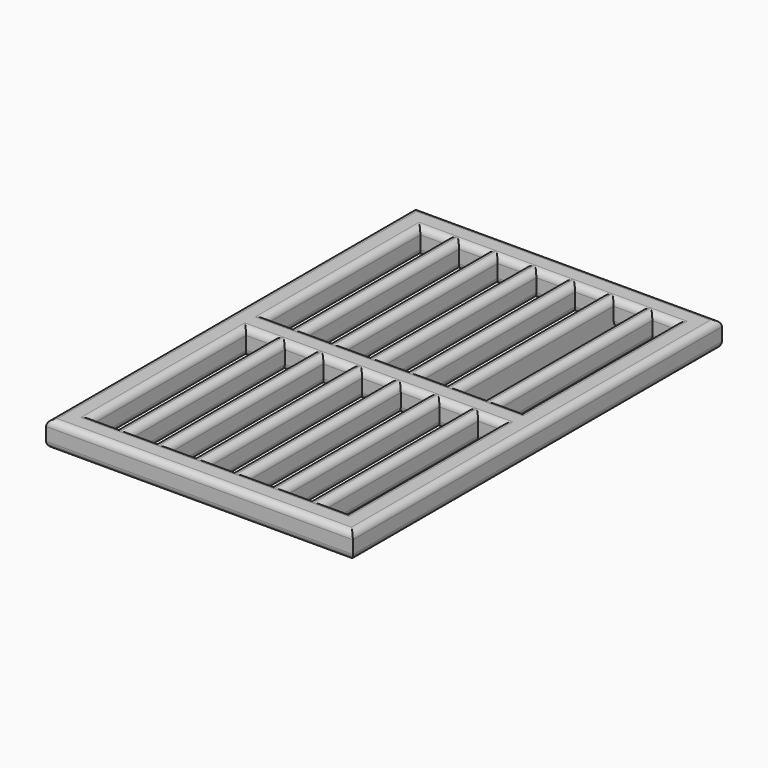
from build123d import *

# Parameters (mm, degrees)
F0_W     = 60.452
F0_H     = 90.932
F0_W_2   = 2.54
F0_H_2   = 37.846
F1_DEPTH = 5.08
F2_R     = 1.26999
F3_R     = 1.26999


# Not quite as in the source:
# - a fillet or chamfer is up to 0.001 mm smaller than in the source, because OpenCascade refuses the exact size


with BuildPart() as f1:
    # F0 (on Top) → F1 (new body)
    with BuildSketch(Plane.XY):
        Rectangle(F0_W, F0_H)
        Polygon((-20.066, -40.386), (-25.146, -40.386), (-25.146, -2.54), (-25.146, 2.54), (-25.146, 40.386), (-20.066, 40.386), (-17.526, 40.386), (-12.446, 40.386), (-9.906, 40.386), (-4.826, 40.386), (-2.286, 40.386), (2.794, 40.386), (5.334, 40.386), (10.414, 40.386), (12.954, 40.386), (18.034, 40.386), (20.574, 40.386), (25.146, 40.386), (25.146, 2.54), (25.146, -2.54), (25.146, -40.386), (20.574, -40.386), (18.034, -40.386), (12.954, -40.386), (10.414, -40.386), (5.334, -40.386), (2.794, -40.386), (-2.286, -40.386), (-4.826, -40.386), (-9.906, -40.386), (-12.446, -40.386), (-17.526, -40.386), align=None, mode=Mode.SUBTRACT)
        Polygon((-25.146, 2.54), (-25.146, -2.54), (-20.066, -2.54), (-17.526, -2.54), (-12.446, -2.54), (-9.906, -2.54), (-4.826, -2.54), (-2.286, -2.54), (2.794, -2.54), (5.334, -2.54), (10.414, -2.54), (12.954, -2.54), (18.034, -2.54), (20.574, -2.54), (25.146, -2.54), (25.146, 2.54), (20.574, 2.54), (18.034, 2.54), (12.954, 2.54), (10.414, 2.54), (5.334, 2.54), (2.794, 2.54), (-2.286, 2.54), (-4.826, 2.54), (-9.906, 2.54), (-12.446, 2.54), (-17.526, 2.54), (-20.066, 2.54), align=None)
        with Locations((-18.796, -21.463)):
            Rectangle(F0_W_2, F0_H_2)
        with Locations((-11.176, -21.463)):
            Rectangle(F0_W_2, F0_H_2)
        with Locations((-3.556, -21.463)):
            Rectangle(F0_W_2, F0_H_2)
        with Locations((4.064, -21.463)):
            Rectangle(F0_W_2, F0_H_2)
        with Locations((11.684, -21.463)):
            Rectangle(F0_W_2, F0_H_2)
        with Locations((19.304, -21.463)):
            Rectangle(F0_W_2, F0_H_2)
        with Locations((19.304, 21.463)):
            Rectangle(F0_W_2, F0_H_2)
        with Locations((11.684, 21.463)):
            Rectangle(F0_W_2, F0_H_2)
        with Locations((4.064, 21.463)):
            Rectangle(F0_W_2, F0_H_2)
        with Locations((-3.556, 21.463)):
            Rectangle(F0_W_2, F0_H_2)
        with Locations((-11.176, 21.463)):
            Rectangle(F0_W_2, F0_H_2)
        with Locations((-18.796, 21.463)):
            Rectangle(F0_W_2, F0_H_2)
    extrude(amount=F1_DEPTH)

    # F2 (radius 1.27 in the source; OpenCascade refuses exactly that, so slightly less here)
    f2_edges = [f1.edges().sort_by_distance(p)[0] for p in [
        (-20.066, 21.463, 5.08),
        (-22.606, 40.386, 5.08),
        (-25.146, 21.463, 5.08),
        (-22.606, 2.54, 5.08),
        (-17.526, 21.463, 5.08),
        (-12.446, 21.463, 5.08),
        (-14.986, 40.386, 5.08),
        (-14.986, 2.54, 5.08),
        (-7.366, 2.54, 5.08),
        (-4.826, 21.463, 5.08),
        (-9.906, 21.463, 5.08),
        (-7.366, 40.386, 5.08),
        (-2.286, 21.463, 5.08),
        (2.794, 21.463, 5.08),
        (0.254, 40.386, 5.08),
        (0.254, 2.54, 5.08),
        (5.334, 21.463, 5.08),
        (7.874, 2.54, 5.08),
        (10.414, 21.463, 5.08),
        (7.874, 40.386, 5.08),
        (12.954, 21.463, 5.08),
        (18.034, 21.463, 5.08),
        (15.494, 2.54, 5.08),
        (15.494, 40.386, 5.08),
        (22.86, 40.386, 5.08),
        (25.146, 21.463, 5.08),
        (20.574, 21.463, 5.08),
        (22.86, 2.54, 5.08),
        (25.146, -21.463, 5.08),
        (20.574, -21.463, 5.08),
        (22.86, -2.54, 5.08),
        (22.86, -40.386, 5.08),
        (15.494, -40.386, 5.08),
        (18.034, -21.463, 5.08),
        (12.954, -21.463, 5.08),
        (15.494, -2.54, 5.08),
        (7.874, -2.54, 5.08),
        (5.334, -21.463, 5.08),
        (10.414, -21.463, 5.08),
        (7.874, -40.386, 5.08),
        (-2.286, -21.463, 5.08),
        (2.794, -21.463, 5.08),
        (0.254, -40.386, 5.08),
        (0.254, -2.54, 5.08),
        (-4.826, -21.463, 5.08),
        (-9.906, -21.463, 5.08),
        (-7.366, -2.54, 5.08),
        (-7.366, -40.386, 5.08),
        (-14.986, -40.386, 5.08),
        (-14.986, -2.54, 5.08),
        (-17.526, -21.463, 5.08),
        (-12.446, -21.463, 5.08),
        (-30.226, 0, 5.08),
        (0, -45.466, 5.08),
        (30.226, 0, 5.08),
        (0, 45.466, 5.08),
        (-25.146, -21.463, 5.08),
        (-22.606, -2.54, 5.08),
        (-20.066, -21.463, 5.08),
        (-22.606, -40.386, 5.08),
    ]]
    fillet(f2_edges, radius=F2_R)

    # F3 (radius 1.27 in the source; OpenCascade refuses exactly that, so slightly less here)
    f3_edges = [f1.edges().sort_by_distance(p)[0] for p in [
        (25.146, 21.463, 0),
        (20.574, 21.463, 0),
        (18.034, 21.463, 0),
        (10.414, 21.463, 0),
        (5.334, 21.463, 0),
        (2.794, 21.463, 0),
        (-2.286, 21.463, 0),
        (-4.826, 21.463, 0),
        (-9.906, 21.463, 0),
        (-12.446, 21.463, 0),
        (-17.526, 21.463, 0),
        (-20.066, 21.463, 0),
        (-25.146, 21.463, 0),
        (-14.986, 40.386, 0),
        (-7.366, 40.386, 0),
        (0.254, 40.386, 0),
        (7.874, 40.386, 0),
        (15.494, 40.386, 0),
        (22.86, 40.386, 0),
        (22.86, 2.54, 0),
        (-22.606, 40.386, 0),
        (15.494, 2.54, 0),
        (7.874, 2.54, 0),
        (0.254, 2.54, 0),
        (-7.366, 2.54, 0),
        (-14.986, 2.54, 0),
        (-22.606, 2.54, 0),
        (-25.146, -21.463, 0),
        (-20.066, -21.463, 0),
        (-17.526, -21.463, 0),
        (-12.446, -21.463, 0),
        (-9.906, -21.463, 0),
        (-4.826, -21.463, 0),
        (-2.286, -21.463, 0),
        (2.794, -21.463, 0),
        (5.334, -21.463, 0),
        (10.414, -21.463, 0),
        (12.954, -21.463, 0),
        (18.034, -21.463, 0),
        (20.574, -21.463, 0),
        (25.146, -21.463, 0),
        (22.86, -2.54, 0),
        (15.494, -2.54, 0),
        (7.874, -2.54, 0),
        (0.254, -2.54, 0),
        (-7.366, -2.54, 0),
        (-14.986, -2.54, 0),
        (-22.606, -2.54, 0),
        (-22.606, -40.386, 0),
        (-14.986, -40.386, 0),
        (-7.366, -40.386, 0),
        (0.254, -40.386, 0),
        (7.874, -40.386, 0),
        (15.494, -40.386, 0),
        (22.86, -40.386, 0),
        (30.226, 0, 0),
        (-30.226, 0, 0),
        (0, -45.466, 0),
        (0, 45.466, 0),
    ]]
    fillet(f3_edges, radius=F3_R)


solid = f1.part
